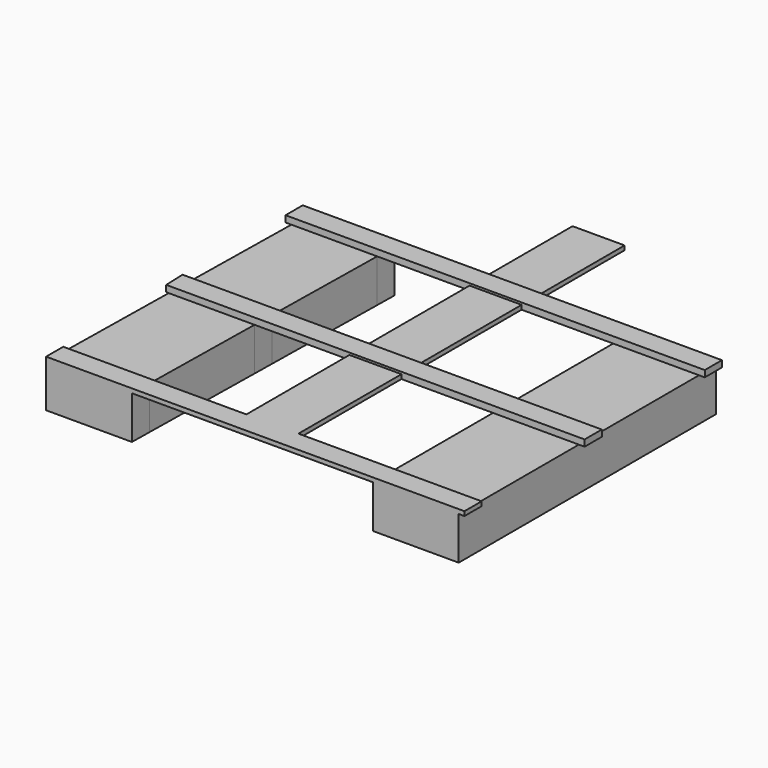
from build123d import *

# Parameters (mm, degrees)
F1_DEPTH = 2
F3_DEPTH = 2
F4_DEPTH = 3
F5_DEPTH = 2
F6_W     = 40
F6_H     = 10
F6_H_2   = 60
F7_DEPTH = 20


with BuildPart() as f1:
    # F0 (on Top) → F1 (new body)
    with BuildSketch(Plane.XY):
        Polygon((-12.130910923, 0), (0, 0), (12.130910923, 0), (12.130910923, 200), (-12.130910923, 200), align=None)
    extrude(amount=F1_DEPTH)

    # F2 (on Top) → F3 (join)
    with BuildSketch(Plane.XY):
        Polygon((-97.5, 0), (0, 0), (97.5, 0), (97.5, 10), (-97.5, 10), align=None)
        Polygon((-97.5, 70), (0, 70), (97.5, 70), (97.5, 80), (-97.8855118155, 80), align=None)
        Polygon((-97.8855118155, 140), (0, 140), (97.5, 140), (97.5, 150), (-97.8855118155, 150), align=None)
    extrude(amount=F3_DEPTH)

    # F2 (on Top) → F4 (join)
    with BuildSketch(Plane.XY):
        Polygon((-97.5, 70), (0, 70), (97.5, 70), (97.5, 80), (-97.8855118155, 80), align=None)
        Polygon((-97.8855118155, 140), (0, 140), (97.5, 140), (97.5, 150), (-97.8855118155, 150), align=None)
    extrude(amount=F4_DEPTH)

    # F2 (on Top) → F5 (join)
    with BuildSketch(Plane.XY):
        Polygon((-97.5, 0), (0, 0), (97.5, 0), (97.5, 10), (-97.5, 10), align=None)
        Polygon((-97.5, 70), (0, 70), (97.5, 70), (97.5, 80), (-97.8855118155, 80), align=None)
        Polygon((-97.8855118155, 140), (0, 140), (97.5, 140), (97.5, 150), (-97.8855118155, 150), align=None)
    extrude(amount=F5_DEPTH)

    # F6 (on face) → F7 (join)
    with BuildSketch(Plane(origin=(0, 0, 0), x_dir=(1, 0, 0), z_dir=(0, 0, -1))):
        Polygon((-57.4945055695, 0), (-97.5, 0), (-97.3342470533, -10), (-57.3287526228, -10), align=None)
        Polygon((-57.3287526228, -10), (-97.3342470533, -10), (-96.3397293732, -70), (-56.3342349427, -70), align=None)
        with Locations((74.8154554615, -5)):
            Rectangle(F6_W, F6_H)
        Polygon((-56.3342349427, -70), (-96.3397293732, -70), (-96.1739764266, -80), (-56.168481996, -80), align=None)
        with Locations((74.8154554615, -40)):
            Rectangle(F6_W, F6_H_2)
        Polygon((-56.168481996, -80), (-96.1739764266, -80), (-95.1794587465, -140), (-55.173964316, -140), align=None)
        with Locations((74.8154554615, -75)):
            Rectangle(F6_W, F6_H)
        Polygon((-55.173964316, -140), (-95.1794587465, -140), (-95.0137057998, -150), (-55.0082113693, -150), align=None)
        with Locations((74.8154554615, -110)):
            Rectangle(F6_W, F6_H_2)
        with Locations((74.8154554615, -145)):
            Rectangle(F6_W, F6_H)
    extrude(amount=F7_DEPTH)


solid = f1.part
